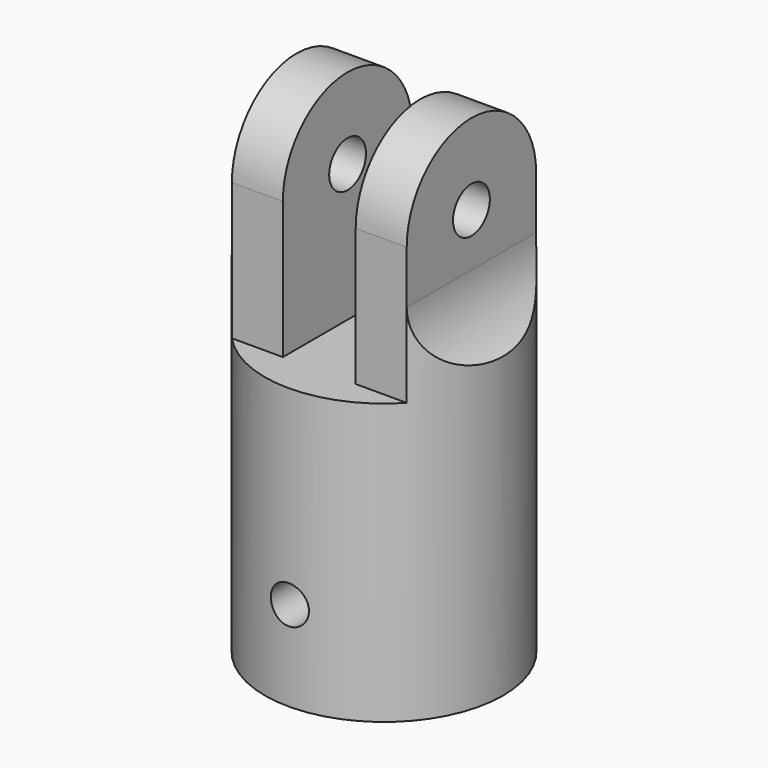
from build123d import *

# Parameters (mm, degrees)
F0_R          = 10.795
F0_R_2        = 6.4897
F1_DEPTH      = 20.32
F2_R          = 10.795
F3_DEPTH      = 5.08
F4_W          = 4.6222759372
F4_H          = 14.661224488
F5_DEPTH      = 12.4206
F6_R          = 1.7272
F7_DEPTH      = 10.796
F7_DEPTH_BACK = 25.4
F9_DEPTH      = 4.6222759372
F10_R         = 7.330612244
F11_DEPTH     = 4.6222759372
F12_R         = 2.0828
F13_DEPTH     = 18.7202760372
F14_T4_DEPTH  = 14.661224488
F14_S5_R      = 10.795
F14_T6_DEPTH  = 11
F14_T10_DEPTH = 14.661224488
F14_S11_R     = 10.795
F14_T12_DEPTH = 11
F15_R         = 1.27


# Not quite as in the source:
# - a fillet or chamfer that OpenCascade refuses, or shapes differently, is made with other operations: its cross-section is extruded or revolved along the edge and cut away or added


with BuildPart() as f1:
    # F0 (on Top) → F1 (new body)
    with BuildSketch(Plane.XY):
        Circle(F0_R)
        Circle(F0_R_2, mode=Mode.SUBTRACT)
    extrude(amount=F1_DEPTH)

    # F2 (on face) → F3 (join)
    with BuildSketch(Plane.XY.offset(20.32)):
        Circle(F2_R)
    extrude(amount=F3_DEPTH)

    # F4 (on face) → F5 (join)
    with BuildSketch(Plane.XY.offset(25.4)):
        with Locations((-5.6131379686, 0)):
            Rectangle(F4_W, F4_H)
        with Locations((5.6131379686, 0)):
            Rectangle(F4_W, F4_H)
    extrude(amount=F5_DEPTH)

    # F6 (on Front) → F7 (cut, two sides)
    with BuildSketch(Plane.XZ) as f7_sk:
        with Locations((0, 8.128)):
            Circle(F6_R)
    extrude(amount=F7_DEPTH, mode=Mode.SUBTRACT)
    extrude(f7_sk.sketch, amount=-F7_DEPTH_BACK, mode=Mode.SUBTRACT)

    # F8 (on face) → F9 (join, through all)
    with BuildSketch(Plane(origin=(3.302, 0, 0), x_dir=(0, -1, 0), z_dir=(-1, 0, 0))):
        with BuildLine():
            Line((-7.330612244, 37.8206), (7.330612244, 37.8206))
            ThreePointArc((7.330612244, 37.8206), (0, 45.151212244), (-7.330612244, 37.8206))
        make_face()
    extrude(amount=-F9_DEPTH)

    # F10 (on face) → F11 (join, through all)
    with BuildSketch(Plane(origin=(-7.9242759372, 0, 0), x_dir=(0, -1, 0), z_dir=(-1, 0, 0))):
        with Locations((0, 37.8206)):
            Circle(F10_R)
    extrude(amount=-F11_DEPTH)

    # F12 (on face) → F13 (cut, through all)
    with BuildSketch(Plane(origin=(-7.9242759372, 0, 0), x_dir=(0, -1, 0), z_dir=(-1, 0, 0))):
        with Locations((0, 37.8206)):
            Circle(F12_R)
    extrude(amount=-F13_DEPTH, mode=Mode.SUBTRACT)

    # F14: fillet of radius 7.62 on 2 edges, made by hand


with BuildPart() as f14_tool2:
    # F14_s3 → F14_t4 (new body)
    with BuildSketch(Plane.XZ.offset(7.330612244)):
        with BuildLine():
            ThreePointArc((15.5442759372, 25.4), (10.1561222645, 27.6318463274), (7.9242759372, 33.02))
            Line((7.9242759372, 33.02), (7.9242759372, 25.4))
            Line((7.9242759372, 25.4), (15.5442759372, 25.4))
        make_face()
    extrude(amount=-F14_T4_DEPTH)

    # F14_s5 → F14_t6 (intersect, symmetric)
    with BuildSketch(Plane.XY.offset(29.2)):
        Circle(F14_S5_R)
    extrude(amount=F14_T6_DEPTH, both=True, mode=Mode.INTERSECT)


with BuildPart() as f1_1:
    add(f1.part)

    # F14_t1: union F14_tool2
    add(f14_tool2.part)


with BuildPart() as f14_tool8:
    # F14_s9 → F14_t10 (new body)
    with BuildSketch(Plane.XZ.offset(-7.330612244)):
        with BuildLine():
            ThreePointArc((-15.5442759372, 25.4), (-10.1561222645, 27.6318463274), (-7.9242759372, 33.02))
            Line((-7.9242759372, 33.02), (-7.9242759372, 25.4))
            Line((-7.9242759372, 25.4), (-15.5442759372, 25.4))
        make_face()
    extrude(amount=F14_T10_DEPTH)

    # F14_s11 → F14_t12 (intersect, symmetric)
    with BuildSketch(Plane.XY.offset(29.2)):
        Circle(F14_S11_R)
    extrude(amount=F14_T12_DEPTH, both=True, mode=Mode.INTERSECT)


with BuildPart() as f1_2:
    add(f1_1.part)

    # F14_t7: union F14_tool8
    add(f14_tool8.part)

    # F15
    f15_edges = [f1_2.edges().sort_by_distance(p)[0] for p in [
        (-6.4897, 0, 0),
    ]]
    fillet(f15_edges, radius=F15_R)


solid = f1_2.part
